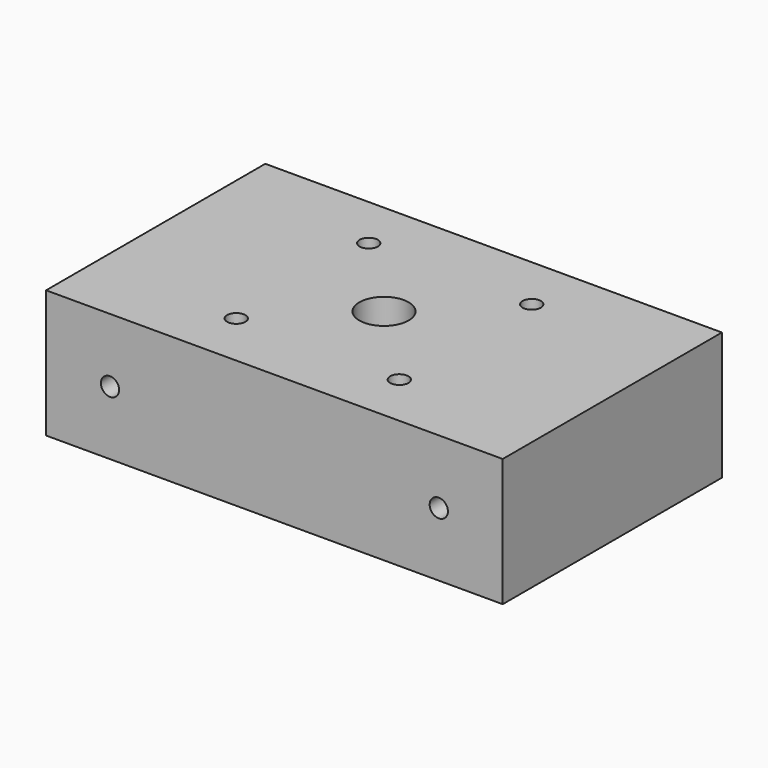
from build123d import *

# Parameters (mm, degrees)
F0_W     = 50
F0_H     = 30
F1_DEPTH = 14
F3_D     = 11
F5_D     = 2
F7_D     = 2
F8_R     = 5.5
F8_R_2   = 2.7
F9_DEPTH = 8


# Not quite as in the source:
# - a feature names something its author has since deleted; it is built from what else it names


with BuildPart() as f1:
    # F0 (on Top) → F1 (new body)
    with BuildSketch(Plane.XY):
        Rectangle(F0_W, F0_H)
    extrude(amount=F1_DEPTH)

    # F3 (through all)
    with Locations(Plane.XY.offset(14)):
        with Locations((0, 0)):
            Hole(F3_D / 2)

    # F5 (through all)
    with Locations(Plane.XY.offset(14)):
        with Locations((-8.9121767002, 9.0478232998), (9.0478232998, 8.9121767002), (8.9121767002, -9.0478232998), (-9.0478232998, -8.9121767002)):
            Hole(F5_D / 2)

    # F7 (through all)
    with Locations(Plane.XZ.offset(15)):
        with Locations((18, 7), (-18, 7)):
            Hole(F7_D / 2)

    # F8 (on face) → F9 (join)
    with BuildSketch(Plane.XY.offset(14)):
        Circle(F8_R)
        Circle(F8_R_2, mode=Mode.SUBTRACT)
    extrude(amount=-F9_DEPTH)


solid = f1.part
